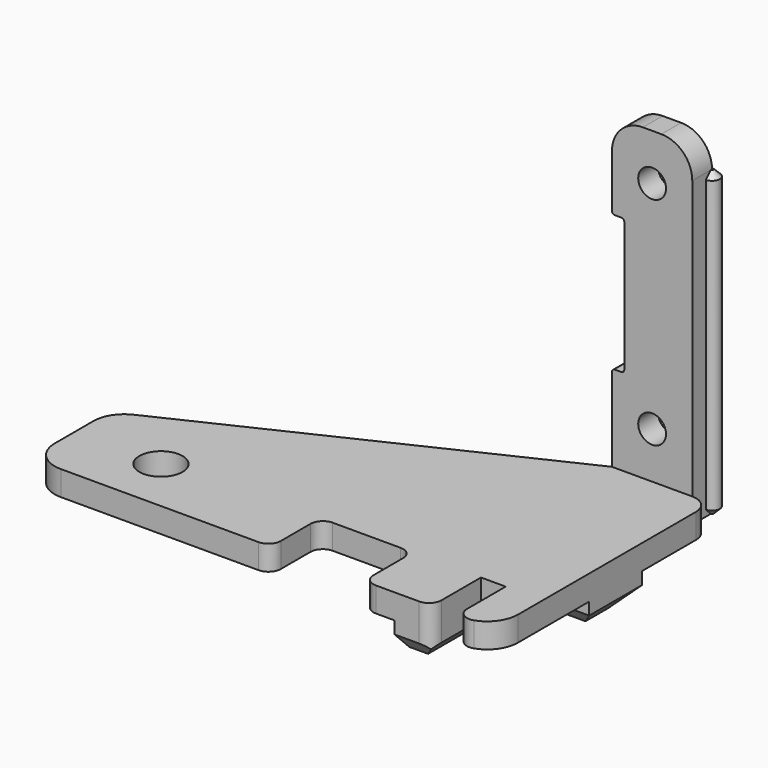
from build123d import *

# Parameters (mm, degrees)
F0_R      = 3.5
F1_DEPTH  = 4
F0_W      = 13
F0_H      = 4
F2_DEPTH  = 54
F3_R      = 5
F4_W      = 6.0393586755
F4_H      = 4
F5_DEPTH  = 5
F6_SIZE   = 3
F4_R      = 1.25
F7_DEPTH  = 49
F8_SIZE   = 1
F9_SIZE   = 1
F10_R     = 2.25
F11_DEPTH = 5
F12_R     = 2
F13_W     = 2
F13_H     = 22
F14_DEPTH = 5
F15_R     = 0.5


with BuildPart() as f1:
    # F0 (on Top) → F1 (new body)
    with BuildSketch(Plane.XY):
        with BuildLine():
            ThreePointArc((0, 5), (1.4644660941, 1.4644660941), (5, 0))
            Line((5, 0), (39, 0))
            Line((39, 0), (39, 10))
            Line((39, 10), (54, 10))
            Line((54, 10), (54, 0))
            Line((54, 0), (65, 0))
            Line((65, 0), (65, 10))
            Line((65, 10), (69, 10))
            Line((69, 10), (69, 0))
            Line((69, 0), (70, 0))
            ThreePointArc((70, 0), (73.5355339059, 1.4644660941), (75, 5))
            Line((75, 5), (75, 41))
            ThreePointArc((75, 41), (74.1213203436, 43.1213203436), (72, 44))
            Line((72, 44), (59, 44))
            Line((59, 44), (2.8562777384, 17.3555216386))
            ThreePointArc((2.8562777384, 17.3555216386), (0.7739728285, 15.5106003536), (0, 12.8383925874))
            Line((0, 12.8383925874), (0, 5))
        make_face()
        with Locations((14, 9)):
            Circle(F0_R, mode=Mode.SUBTRACT)
    extrude(amount=F1_DEPTH)

    # F0 (on Top) → F2 (join)
    with BuildSketch(Plane.XY):
        with Locations((65.5, 46)):
            Rectangle(F0_W, F0_H)
    extrude(amount=F2_DEPTH)

    # F3
    f3_edges = [f1.edges().sort_by_distance(p)[0] for p in [
        (72, 46, 54),
        (59, 46, 54),
    ]]
    fillet(f3_edges, radius=F3_R)

    # F4 (on face) → F5 (join)
    with BuildSketch(Plane.XY):
        Polygon((29.5861130485, 30.0408672094), (7.1886969879, 19.3925328106), (59, 19.3925328106), (59, 0), (65, 0), (65, 10), (65.0393586755, 10), (65.0393586755, 19.3925328106), (75, 19.3925328106), (75, 30.0408672094), (65.0393586755, 30.0408672094), (65.0393586755, 44), (59, 44), (59, 30.0408672094), align=None)
        with Locations((62.0196793377, 46)):
            Rectangle(F4_W, F4_H)
    extrude(amount=-F5_DEPTH)

    # F6 (call 1 of 4: OpenCascade refuses the feature's edges together)
    f6_edges = [f1.edges().sort_by_distance(p)[0] for p in [
        (62.019679, 48, -5),
        (75, 24.7167, -5),
        (70.019679, 30.040867, -5),
        (70.019679, 19.392533, -5),
        (65.039359, 39.020434, -5),
        (65.039359, 14.696266, -5),
    ]]
    chamfer(f6_edges, length=F6_SIZE)

    # F6#2 (call 2 of 4)
    f6_2_edges = [f1.edges().sort_by_distance(p)[0] for p in [
        (62, 0, -5),
    ]]
    chamfer(f6_2_edges, length=F6_SIZE)

    # F6#3 (call 3 of 4)
    f6_3_edges = [f1.edges().sort_by_distance(p)[0] for p in [
        (44.293057, 30.040867, -5),
    ]]
    chamfer(f6_3_edges, length=F6_SIZE)

    # F6#4 (call 4 of 4)
    f6_4_edges = [f1.edges().sort_by_distance(p)[0] for p in [
        (33.094348, 19.392533, -5),
    ]]
    chamfer(f6_4_edges, length=F6_SIZE)

    # F4 (on face) → F7 (join)
    with BuildSketch(Plane.XY):
        with Locations((72, 48)):
            Circle(F4_R)
    extrude(amount=F7_DEPTH)

    # F8
    f8_edges = [f1.edges().sort_by_distance(p)[0] for p in [
        (72.883883, 48.883883, 49),
    ]]
    chamfer(f8_edges, length=F8_SIZE)

    # F9
    f9_edges = [f1.edges().sort_by_distance(p)[0] for p in [
        (72.883883, 48.883883, 0),
    ]]
    chamfer(f9_edges, length=F9_SIZE)

    # F10 (on face) → F11 (cut)
    with BuildSketch(Plane(origin=(0, 48, 0), x_dir=(-1, 0, 0), z_dir=(0, 1, 0))):
        with Locations((-65.5, 11.5)):
            Circle(F10_R)
        with Locations((-65.5, 46.5)):
            Circle(F10_R)
    extrude(amount=-F11_DEPTH, mode=Mode.SUBTRACT)

    # F12
    f12_edges = [f1.edges().sort_by_distance(p)[0] for p in [
        (54, 10, 2),
        (54, 0, 2),
        (39, 10, 2),
        (39, 0, 2),
        (65, 0, 1),
        (69, 0, 2),
    ]]
    fillet(f12_edges, radius=F12_R)

    # F13 (on face) → F14 (cut)
    with BuildSketch(Plane(origin=(0, 48, 0), x_dir=(-1, 0, 0), z_dir=(0, 1, 0))):
        with Locations((-60, 29)):
            Rectangle(F13_W, F13_H)
    extrude(amount=-F14_DEPTH, mode=Mode.SUBTRACT)

    # F15
    f15_edges = [f1.edges().sort_by_distance(p)[0] for p in [
        (59, 46, 40),
        (59, 46, 18),
        (61, 46, 18),
        (61, 46, 40),
    ]]
    fillet(f15_edges, radius=F15_R)


solid = f1.part
